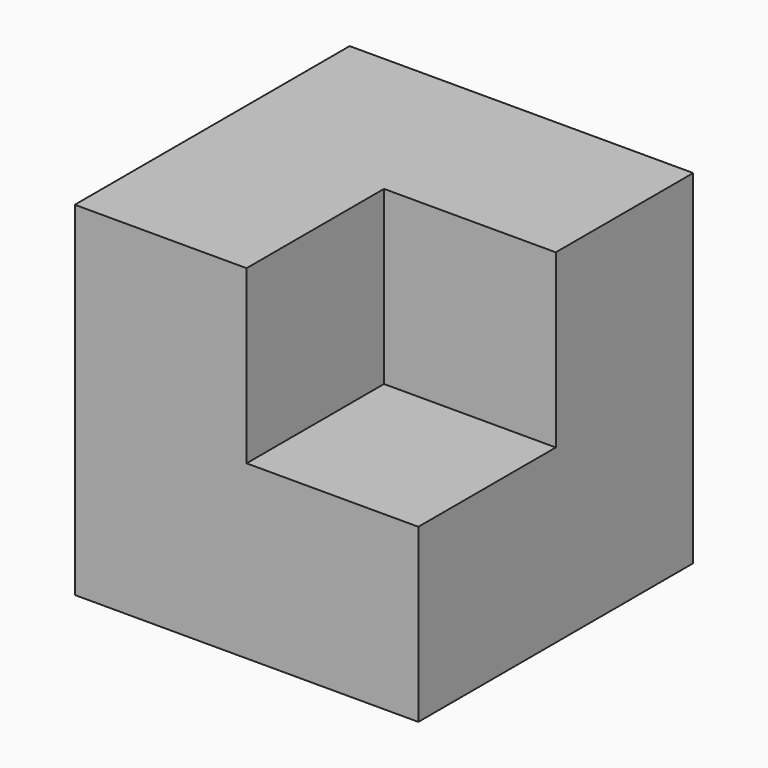
from build123d import *

# Parameters (mm, degrees)
F0_W     = 50.8
F0_H     = 50.8
F1_DEPTH = 50.8
F2_W     = 25.4
F2_H     = 25.4
F3_DEPTH = 25.4


# Not quite as in the source:
# - a feature names something its author has since deleted; it is built from what else it names


with BuildPart() as f1:
    # F0 (on Front) → F1 (new body)
    with BuildSketch(Plane.XZ):
        with Locations((-44.4764100671, 25.4)):
            Rectangle(F0_W, F0_H)
    extrude(amount=F1_DEPTH)

    # F2 (on face) → F3 (cut)
    with BuildSketch(Plane.XZ.offset(50.8)):
        with Locations((-31.7764100671, 38.1)):
            Rectangle(F2_W, F2_H)
    extrude(amount=-F3_DEPTH, mode=Mode.SUBTRACT)


solid = f1.part
